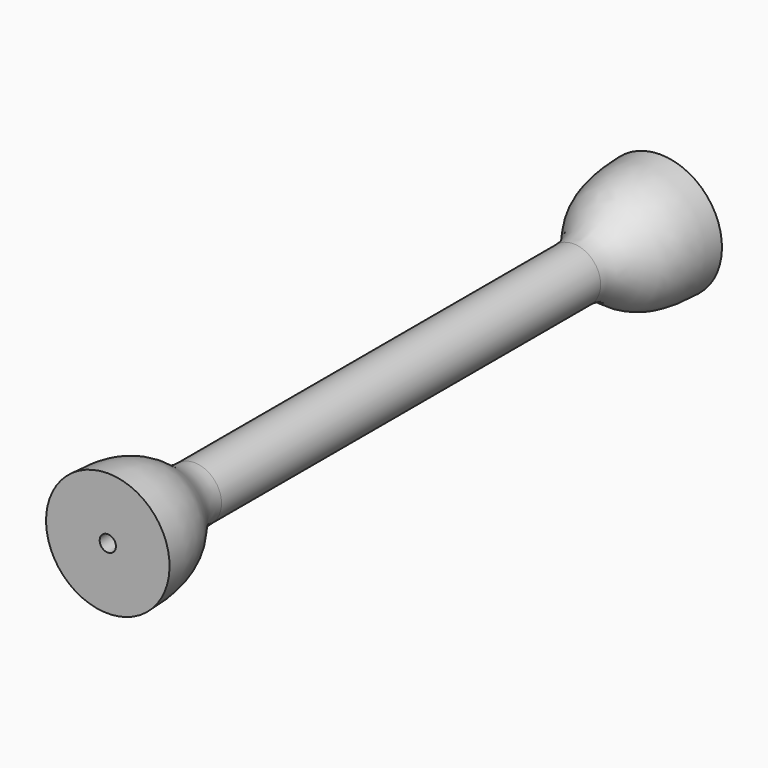
from build123d import *

# Parameters (mm, degrees)
F2_R     = 0.9
F3_DEPTH = 8


with BuildPart() as f1:
    # F0 (on Right) → F1 (revolve)
    with BuildSketch(Plane.YZ):
        with BuildLine():
            Line((0, 5.841069423), (0, 0))
            Line((0, 0), (12, 0))
            Line((12, 0), (12, 2))
            add(Edge.make_bspline(
                [(0, 5.841069423), (0.3497183744, 5.8426503833), (1.3005439266, 5.8382623264), (2.8964802159, 5.7455783673), (4.5870476785, 5.3782777015), (5.9874523646, 4.7970685822), (7.0213600835, 4.1135251272), (7.9242720145, 3.365273981), (8.9405324509, 2.6085376072), (10.1254552113, 2.0890201928), (11.1979079035, 1.9926198646), (11.7889157433, 1.9938020422), (12, 2)],
                knots=[0.0080728178, 0.0080728178, 0.0080728178, 0.0080728178, 1.0595032706, 2.8567052188, 4.7969778976, 6.2186626182, 7.3787538627, 8.5000771421, 9.7368937359, 11.1749138539, 12.3063283312, 12.9431817135, 12.9431817135, 12.9431817135, 12.9431817135], degree=3))
        make_face()
        with BuildLine():
            Line((0, 6.841), (0, 5.841069423))
            add(Edge.make_bspline(
                [(0, 5.841069423), (0.3497183744, 5.8426503833), (1.3005439266, 5.8382623264), (2.8964802159, 5.7455783673), (4.5870476785, 5.3782777015), (5.9874523646, 4.7970685822), (7.0213600835, 4.1135251272), (7.9242720145, 3.365273981), (8.9405324509, 2.6085376072), (10.1254552113, 2.0890201928), (11.1979079035, 1.9926198646), (11.7889157433, 1.9938020422), (12, 2)],
                knots=[0.0080728178, 0.0080728178, 0.0080728178, 0.0080728178, 1.0595032706, 2.8567052188, 4.7969778976, 6.2186626182, 7.3787538627, 8.5000771421, 9.7368937359, 11.1749138539, 12.3063283312, 12.9431817135, 12.9431817135, 12.9431817135, 12.9431817135], degree=3))
            Line((12, 2), (38.25, 2))
            Line((38.25, 2), (38.25, 3))
            Line((38.25, 3), (12, 3))
            add(Edge.make_bspline(
                [(0, 6.841), (8.7633541102, 6.7704077573), (7.4586680881, 3), (12, 3)],
                knots=[0, 0, 0, 0, 12.5997333702, 12.5997333702, 12.5997333702, 12.5997333702], degree=3))
        make_face()
    revolve(axis=Axis((0, 19.125, 0), (0, -1, 0)))

    # F2 (on face) → F3 (cut)
    with BuildSketch(Plane.XZ):
        Circle(F2_R)
    extrude(amount=-F3_DEPTH, mode=Mode.SUBTRACT)

    # F4: F1 across face


with BuildPart() as f1_1:
    add(f1.part)
    add(f1.part.mirror(Plane(origin=(0, 38.25, 0), x_dir=(-1, 0, 0), z_dir=(0, 1, 0))))


solid = f1_1.part
